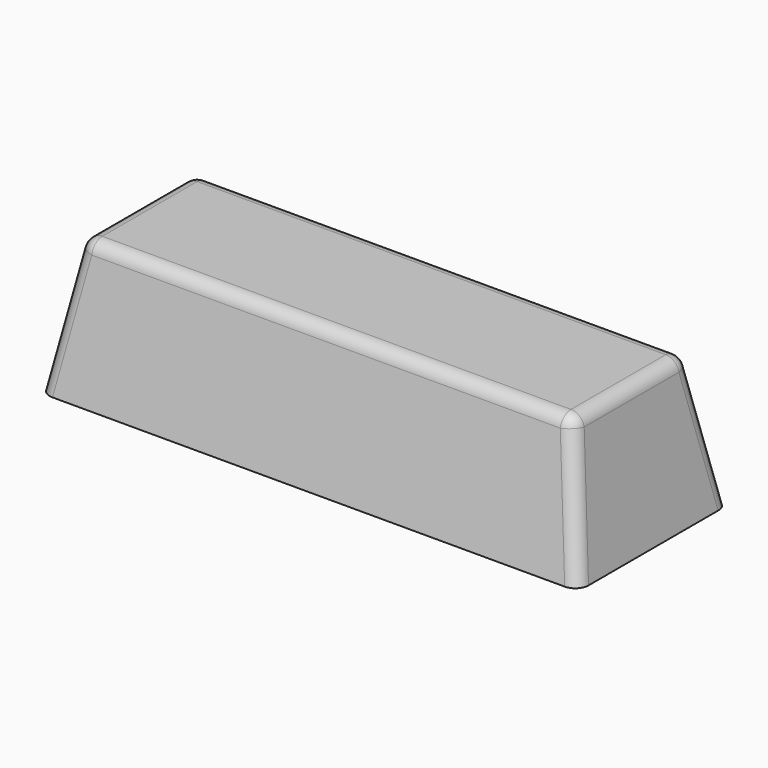
from build123d import *

# Parameters (mm, degrees)
F0_W     = 200
F0_H     = 70
F1_DEPTH = 50
F1_TAPER = 10
F2_R     = 5


with BuildPart() as f1:
    # F0 (on Top) → F1 (new body)
    with BuildSketch(Plane.XY):
        Rectangle(F0_W, F0_H)
    extrude(amount=F1_DEPTH, taper=F1_TAPER)

    # F2
    f2_edges = [f1.edges().sort_by_distance(p)[0] for p in [
        (-91.183651, 0, 50),
        (0, -26.183651, 50),
        (-95.591825, -30.591825, 25),
        (0, 26.183651, 50),
        (91.183651, 0, 50),
        (95.591825, -30.591825, 25),
        (-95.591825, 30.591825, 25),
        (95.591825, 30.591825, 25),
    ]]
    fillet(f2_edges, radius=F2_R)


solid = f1.part
